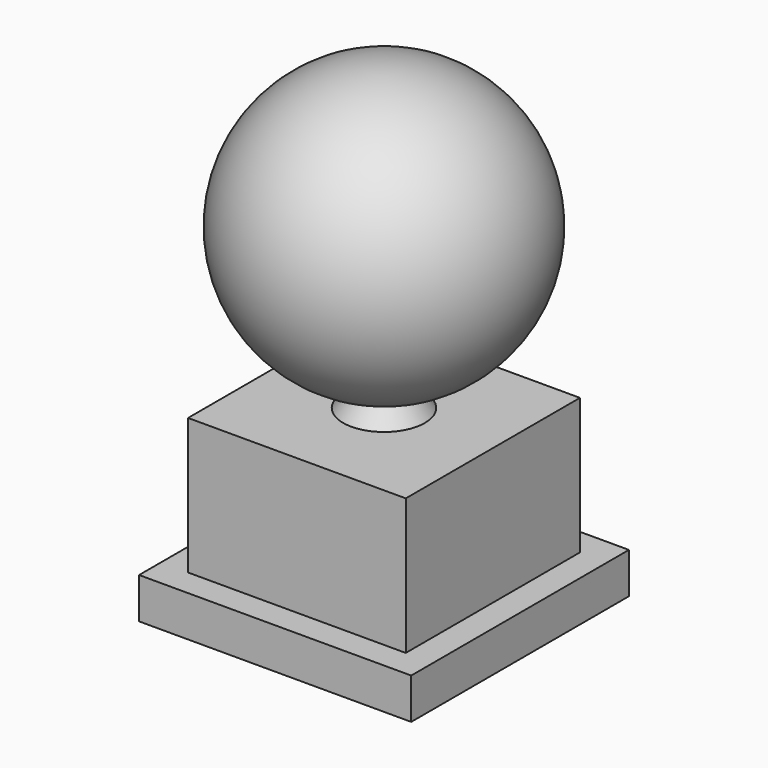
from build123d import *

# Parameters (mm, degrees)
F0_W     = 50.8
F0_H     = 50.8
F1_DEPTH = 7.62
F2_W     = 40.64
F2_H     = 40.64
F3_DEPTH = 25.4
F4_R     = 7.62
F6_R     = 4.445


with BuildPart() as f1:
    # F0 (on Top) → F1 (new body)
    with BuildSketch(Plane.XY):
        Rectangle(F0_W, F0_H)
    extrude(amount=F1_DEPTH)

    # F2 (on face) → F3 (join)
    with BuildSketch(Plane.XY.offset(7.62)):
        Rectangle(F2_W, F2_H)
    extrude(amount=F3_DEPTH)

    # F4 (on face) → F7 section 0
    with BuildSketch(Plane.XY.offset(33.02)):
        Circle(F4_R)
    # F6 (on offset) → F7 section 1
    with BuildSketch(Plane.XY.offset(38.1)):
        Circle(F6_R)
    loft()

    # F9 (on offset) → F10 (revolve)
    with BuildSketch(Plane.YZ):
        with BuildLine():
            Line((0, 37.4538087019), (0, 36.551290824))
            ThreePointArc((0, 36.551290824), (26.302517878, 62.8538087019), (0, 89.1563265799))
            Line((0, 89.1563265799), (0, 88.2538087019))
            Line((0, 88.2538087019), (0, 37.4538087019))
        make_face()
    revolve(axis=Axis((0, 0, 62.8538087019), (0, 0, -1)))


solid = f1.part
